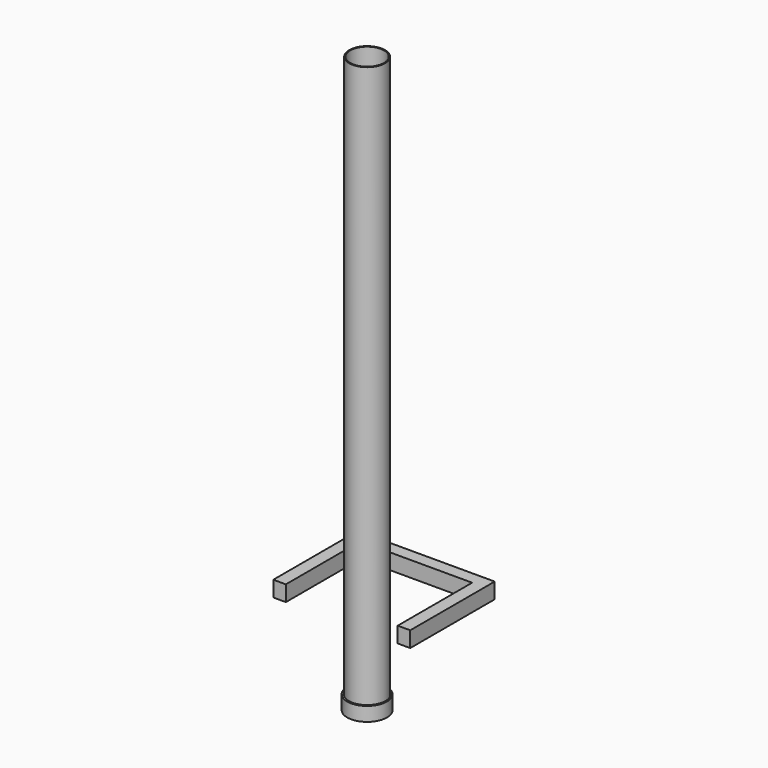
from build123d import *

# Parameters (mm, degrees)
F0_R      = 28.575
F0_R_2    = 26.9875
F1_DEPTH  = 914.4
F2_R      = 24
F3_DEPTH  = 76.2
F5_R      = 31.75
F5_R_2    = 29.21
F6_DEPTH  = 19.05
F4_R      = 31.75
F7_DEPTH  = 3.302
F10_DEPTH = 12.5


with BuildPart() as f1:
    # F0 (on Top) → F1 (new body)
    with BuildSketch(Plane.XY):
        Circle(F0_R)
        Circle(F0_R_2, mode=Mode.SUBTRACT)
    extrude(amount=F1_DEPTH)


with BuildPart() as f3:
    # F2 (on Top) → F3 (new body)
    with BuildSketch(Plane.XY):
        Circle(F2_R)
    extrude(amount=F3_DEPTH)


with BuildPart() as f6:
    # F5 (on Top) → F6 (new body)
    with BuildSketch(Plane.XY):
        Circle(F5_R)
        Circle(F5_R_2, mode=Mode.SUBTRACT)
    extrude(amount=F6_DEPTH)

    # F4 (on Top) → F7 (join)
    with BuildSketch(Plane.XY):
        Circle(F4_R)
    extrude(amount=-F7_DEPTH)


with BuildPart() as f10:
    # F9 (on offset) → F10 (new body, symmetric)
    with BuildSketch(Plane.XY.offset(152.4)):
        Polygon((-89.2200332342, 97.9006469014), (89.2200332342, 97.9006469014), (89.2200332342, -50.5176782608), (109.2200332342, -50.5176782608), (109.2200332342, 117.9006469014), (-109.2200332342, 117.9006469014), (-109.2200332342, -50.5176782608), (-89.2200332342, -50.5176782608), align=None)
    extrude(amount=F10_DEPTH, both=True)


solid = Compound([f1.part, f3.part, f6.part, f10.part])
